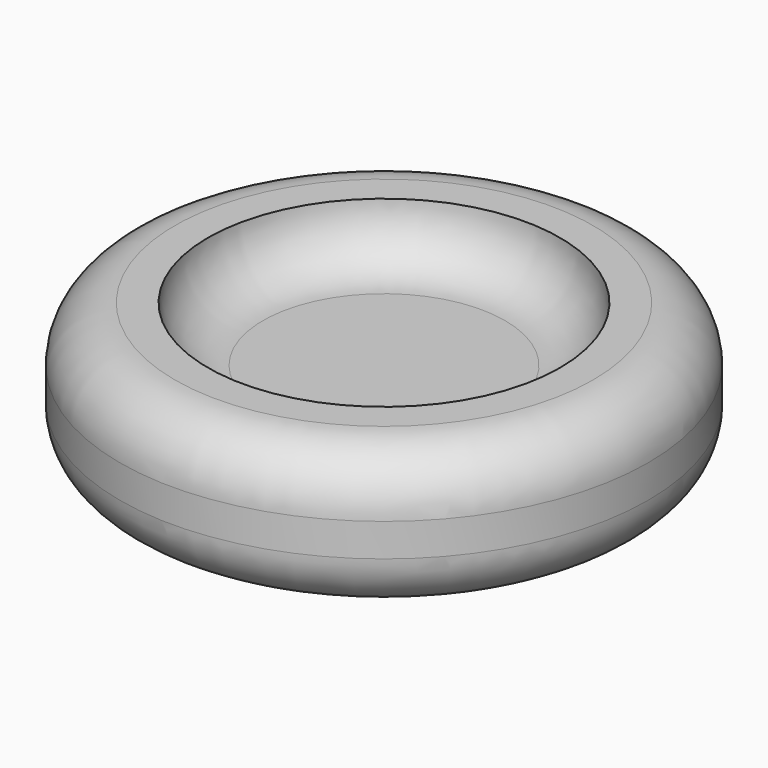
from build123d import *

# Parameters (mm, degrees)
F0_R     = 16
F1_DEPTH = 5
F2_T     = 8


# Not quite as in the source:
# - a fillet or chamfer that OpenCascade refuses, or shapes differently, is made with other operations: its cross-section is extruded or revolved along the edge and cut away or added
# - two fillets or chamfers of one size are made in one step
# - a feature of the source that left no trace in its solid (it failed there, or was rolled back) is left out


with BuildPart() as f1:
    # F0 (on Top) → F1 (new body)
    with BuildSketch(Plane.XY):
        with Locations((-3.0124252662, 6.3863405958)):
            Circle(F0_R)
    extrude(amount=F1_DEPTH)

    # F2
    f2_openings = [f1.faces().sort_by_distance(p)[0] for p in [
        (-3.012425, 6.386341, 5),
    ]]
    offset(amount=F2_T, openings=f2_openings, kind=Kind.INTERSECTION)

    # F3: fillet of radius 5 on 3 edges, made by hand

    # F3_s1 → F3_t2 (revolve)
    with BuildSketch(Plane.XZ.offset(-6.3863405958)):
        with BuildLine():
            ThreePointArc((12.9875747338, 5), (11.5231086397, 1.4644660941), (7.9875747338, 0))
            Line((7.9875747338, 0), (12.9875747338, 0))
            Line((12.9875747338, 0), (12.9875747338, 5))
        make_face()
    revolve(axis=Axis((-3.0124252662, 6.3863405958, 0), (0, 0, 1)))

    # F3_s3 → F3_t4 (revolve, cut)
    with BuildSketch(Plane.XZ.offset(-6.3863405958)):
        with BuildLine():
            ThreePointArc((15.9875747338, 5), (19.5231086397, 3.5355339059), (20.9875747338, 0))
            Line((20.9875747338, 0), (20.9875747338, 5))
            Line((20.9875747338, 5), (15.9875747338, 5))
        make_face()
    revolve(axis=Axis((-3.0124252662, 6.3863405958, 5), (0, 0, -1)), mode=Mode.SUBTRACT)

    # F3_s5 → F3_t6 (revolve, cut)
    with BuildSketch(Plane.XZ.offset(-6.3863405958)):
        with BuildLine():
            ThreePointArc((20.9875747338, -3), (19.5231086397, -6.5355339059), (15.9875747338, -8))
            Line((15.9875747338, -8), (20.9875747338, -8))
            Line((20.9875747338, -8), (20.9875747338, -3))
        make_face()
    revolve(axis=Axis((-3.0124252662, 6.3863405958, -8), (0, 0, -1)), mode=Mode.SUBTRACT)


solid = f1.part
